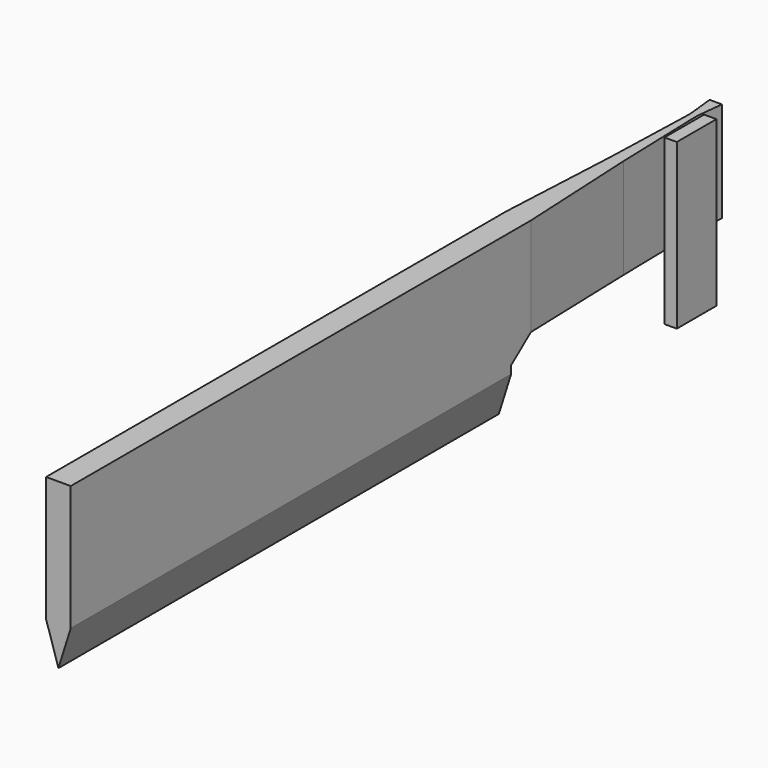
from build123d import *

# Parameters (mm, degrees)
F0_W      = 3
F0_H      = 100
F1_DEPTH  = 20
F2_W      = 1
F2_H      = 4.7696960071
F3_DEPTH  = 100.001
F5_DEPTH  = 20.001
F7_DEPTH  = 7.4319088021
F8_R      = 10
F9_R      = 1.85
F10_DEPTH = 4.9600119411
F11_W     = 1.5
F11_H     = 6.0229186812
F12_DEPTH = 20


# Not quite as in the source:
# - the program builds the solid bodies; features that only make, move or delete a surface that nothing else refers to are left out


with BuildPart() as f1:
    # F0 (on Top) → F1 (new body)
    with BuildSketch(Plane.XY):
        Rectangle(F0_W, F0_H)
    extrude(amount=F1_DEPTH)

    # F2 (on face) → F3 (cut, through all)
    with BuildSketch(Plane.XZ.offset(50)):
        with Locations((-2, 2.3848480035)):
            Rectangle(F2_W, F2_H)
        Polygon((-1.5, 0), (0, 0), (-1.5, 4.7696960071), align=None)
        Polygon((1.5, 4.7696960071), (0, 0), (1.5, 0), align=None)
        with Locations((2, 2.3848480035)):
            Rectangle(F2_W, F2_H)
    extrude(amount=-F3_DEPTH, mode=Mode.SUBTRACT)

    # F4 (on face) → F5 (cut, through all)
    with BuildSketch(Plane.XY.offset(20)):
        Polygon((-1.62, 20), (-1.5, 20), (-0.75, 35), (-0.38, 46.598598361), (-0.75, 50), (-1.62, 50), align=None)
        Polygon((1.62, 20), (1.62, 50), (0.75, 50), (0.38, 46.598598361), (0.75, 35), (1.5, 20), align=None)
    extrude(amount=-F5_DEPTH, mode=Mode.SUBTRACT)

    # F6 (on face) → F7 (cut, through all)
    with BuildSketch(Plane(origin=(0, 0, 0), x_dir=(0, -1, 0), z_dir=(-0.9539392014, 0, -0.3))):
        Polygon((-20, 7.2181625292), (-50.5925305188, 7.2181625292), (-50.5925305188, -0.6273934268), (-17, -0.6273934268), (-17, 5), align=None)
    extrude(amount=-F7_DEPTH, mode=Mode.SUBTRACT)

    # F8
    f8_edges = [f1.edges().sort_by_distance(p)[0] for p in [
        (-0.75, 35, 13.665413),
        (0.75, 35, 13.901277),
        (0.38, 46.598598, 13.843097),
        (-0.38, 46.598598, 13.723593),
    ]]
    fillet(f8_edges, radius=F8_R)

    # F9 (on face) → F10 (cut, through all)
    with BuildSketch(Plane(origin=(-1.8646167189, 0.0594820309, 0), x_dir=(-0.0318841872, -0.9994915701, 0), z_dir=(-0.9994915701, 0.0318841872, 0))):
        with Locations((-43.930772692, 13.7103971598)):
            Circle(F9_R)
    extrude(amount=-F10_DEPTH, mode=Mode.SUBTRACT)


with BuildPart() as f12:
    # F11 (on face) → F12 (new body)
    with BuildSketch(Plane.XY.offset(20)):
        with Locations((1.491804529, 44.2853828522)):
            Rectangle(F11_W, F11_H)
    extrude(amount=-F12_DEPTH)


solid = Compound([f1.part, f12.part])
